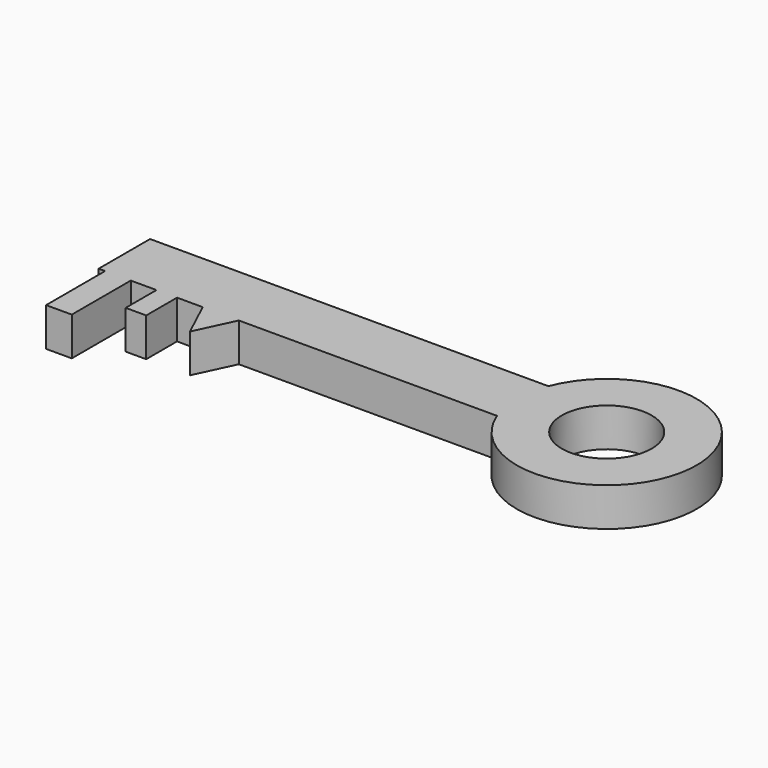
from build123d import *

# Parameters (mm, degrees)
F0_R     = 17.5
F0_W     = 10
F0_H     = 28.6961602334
F0_W_2   = 8
F0_H_2   = 15
F1_DEPTH = 15


# Not quite as in the source:
# - a feature of the source that left no trace in its solid (it failed there, or was rolled back) is left out


with BuildPart() as f1:
    # F0 (on Top) → F1 (new body)
    with BuildSketch(Plane.XY):
        Polygon((122.6644553625, 14.977986814), (122.6644553625, 39.977986814), (-32.3355446375, 39.977986814), (-32.3355446375, 14.977986814), (-29.8321247846, 14.977986814), (-19.8321247846, 14.977986814), (-9.8321247846, 14.977986814), (-1.8321247846, 14.977986814), (8.1678752154, 14.977986814), (22.2149824233, 14.977986814), align=None)
        with BuildLine():
            ThreePointArc((122.6644553625, 14.977986814), (190.356197439, 27.477986814), (122.6644553625, 39.977986814))
            Line((122.6644553625, 39.977986814), (122.6644553625, 14.977986814))
        make_face()
        with Locations((155.356197439, 27.477986814)):
            Circle(F0_R, mode=Mode.SUBTRACT)
        with Locations((-24.8321247846, 0.6299066973)):
            Rectangle(F0_W, F0_H)
        with Locations((-5.8321247846, 7.477986814)):
            Rectangle(F0_W_2, F0_H_2)
        Polygon((15.1678752154, 0), (22.2149824233, 14.977986814), (8.1678752154, 14.977986814), align=None)
    extrude(amount=F1_DEPTH)


solid = f1.part
